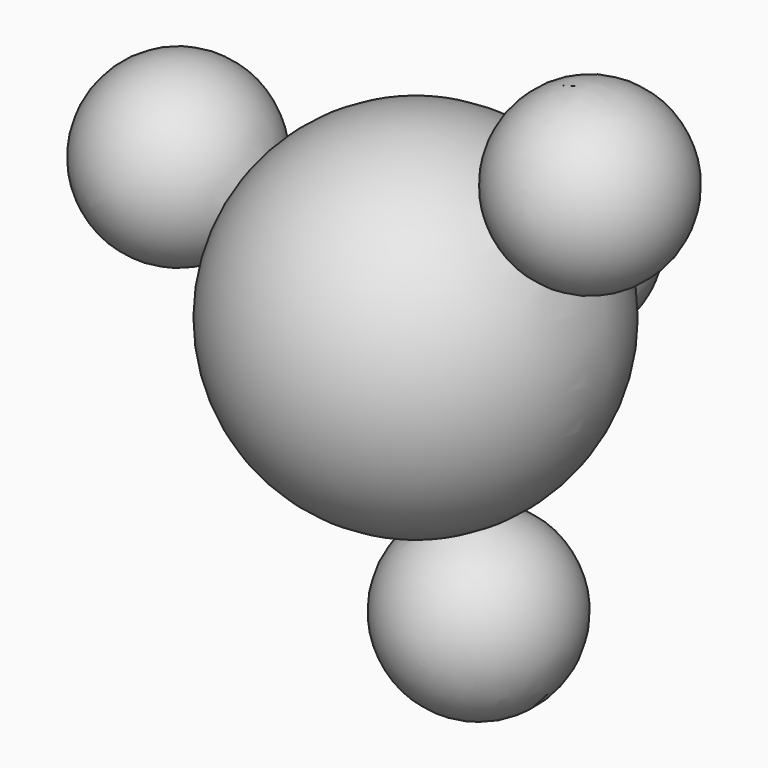
from build123d import *

# Parameters (mm, degrees)
F5_COPIES_COUNT = 3


# Not quite as in the source:
# - a pattern or mirror of a feature is missing from the dataset's text; its kind, count and spacing are read off the source's solid


with BuildPart() as f1:
    # F0 (on Front) → F1 (revolve)
    with BuildSketch(Plane.XZ):
        with BuildLine():
            Line((0, 7), (0, 0))
            Line((0, 0), (0, -7))
            ThreePointArc((0, -7), (7, 0), (0, 7))
        make_face()
    revolve(axis=Axis((0, 0, 3.5), (0, 0, 1)))

    # F4 (on line) → F5 (revolve)
    with BuildSketch(Plane.YZ.offset(7.0336572826)):
        with BuildLine():
            Line((-3.5, 7), (3.5, 7))
            ThreePointArc((3.5, 7), (0, 10.5), (-3.5, 7))
        make_face()
    f5 = revolve(axis=Axis((7.0336572826, 0, 7), (0, -1, 0)))

    # F5_copies: F5 ×3 about axis
    f5_copies_axis = Axis((0, 0, 0), (0, 1, 0))
    for i in range(1, F5_COPIES_COUNT):
        add(f5.rotate(f5_copies_axis, i * 360 / F5_COPIES_COUNT))

    # F7 (on Right) → F8 (revolve)
    with BuildSketch(Plane.YZ):
        with BuildLine():
            ThreePointArc((7.0138228415, -3.4998250146), (10.4788247347, 0), (7.0138228415, 3.4998250146))
            Line((7.0138228415, 3.4998250146), (7.0138228415, -3.4998250146))
        make_face()
    revolve(axis=Axis((0, 7.0138228415, 0), (0, 0, -1)))


solid = f1.part
